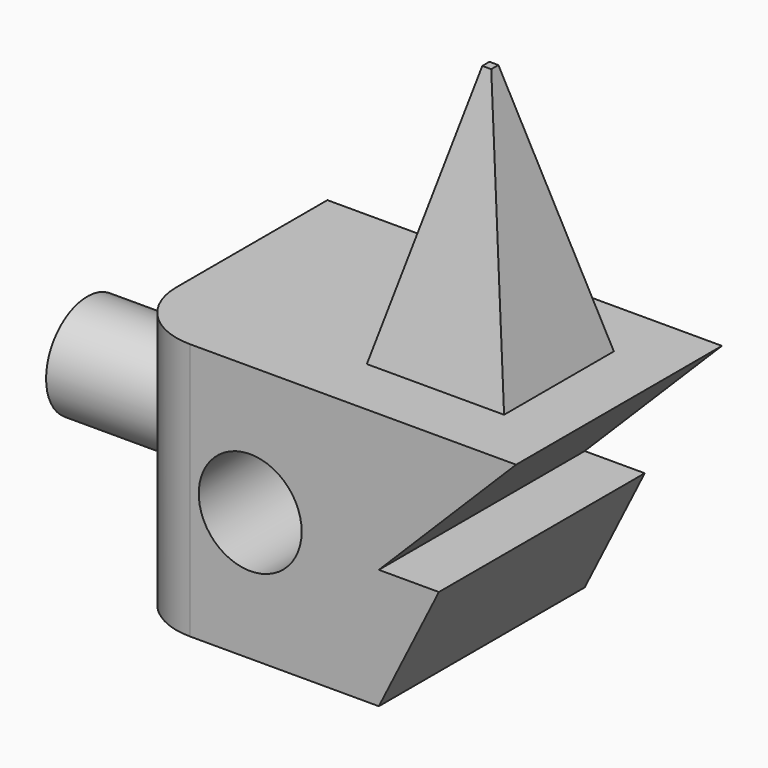
from build123d import *

# Parameters (mm, degrees)
F0_W          = 15
F0_H          = 15
F1_DEPTH      = 15
F3_DEPTH      = 15
F4_R          = 3
F5_DEPTH      = 10
F6_R          = 3
F7_DEPTH      = 8
F8_W          = 8
F8_H          = 8
F9_DEPTH      = 15
F9_TAPER      = 14
F10_R         = 4
F11_TEXT_SIZE = 3.9291926737
F12_DEPTH     = 0.5


# Not quite as in the source:
# - Text() gives the source's letters only with a copy of the font that has no kerning and outlines rounded to 1/6400 em; it was checked with that copy


with BuildPart() as f1:
    # F0 (on Front) → F1 (new body)
    with BuildSketch(Plane.XZ):
        with Locations((7.5, 7.5)):
            Rectangle(F0_W, F0_H)
    extrude(amount=F1_DEPTH)

    # F2 (on face) → F3 (join, through all)
    with BuildSketch(Plane.XZ.offset(15)):
        Polygon((15, 7), (15, 0), (18.5, 7), align=None)
        Polygon((15, 15), (15, 7), (23, 15), align=None)
    extrude(amount=-F3_DEPTH)

    # F4 (on face) → F5 (cut)
    with BuildSketch(Plane.XZ.offset(15)):
        with Locations((7.5, 7.5)):
            Circle(F4_R)
    extrude(amount=-F5_DEPTH, mode=Mode.SUBTRACT)

    # F6 (on face) → F7 (join)
    with BuildSketch(Plane(origin=(0, 0, 0), x_dir=(0, -1, 0), z_dir=(-1, 0, 0))):
        with Locations((7.5, 7.5)):
            Circle(F6_R)
    extrude(amount=F7_DEPTH)

    # F8 (on face) → F9 (join)
    with BuildSketch(Plane.XY.offset(15)):
        with Locations((15.5, -7.5)):
            Rectangle(F8_W, F8_H)
    extrude(amount=F9_DEPTH, taper=F9_TAPER)

    # F10
    f10_edges = [f1.edges().sort_by_distance(p)[0] for p in [
        (0, -15, 7.5),
    ]]
    fillet(f10_edges, radius=F10_R)

    # F11 (on face) → F12 (cut)
    with BuildSketch(Plane(origin=(0, 0, 0), x_dir=(-1, 0, 0), z_dir=(0, 1, 0))):
        with Locations((-14.1114633558, 11.2546886294)):
            Text('Blupsi', F11_TEXT_SIZE, font='Arimo', font_style=FontStyle.BOLD, text_align=(TextAlign.LEFT, TextAlign.BOTTOM))
    extrude(amount=-F12_DEPTH, mode=Mode.SUBTRACT)


solid = f1.part
